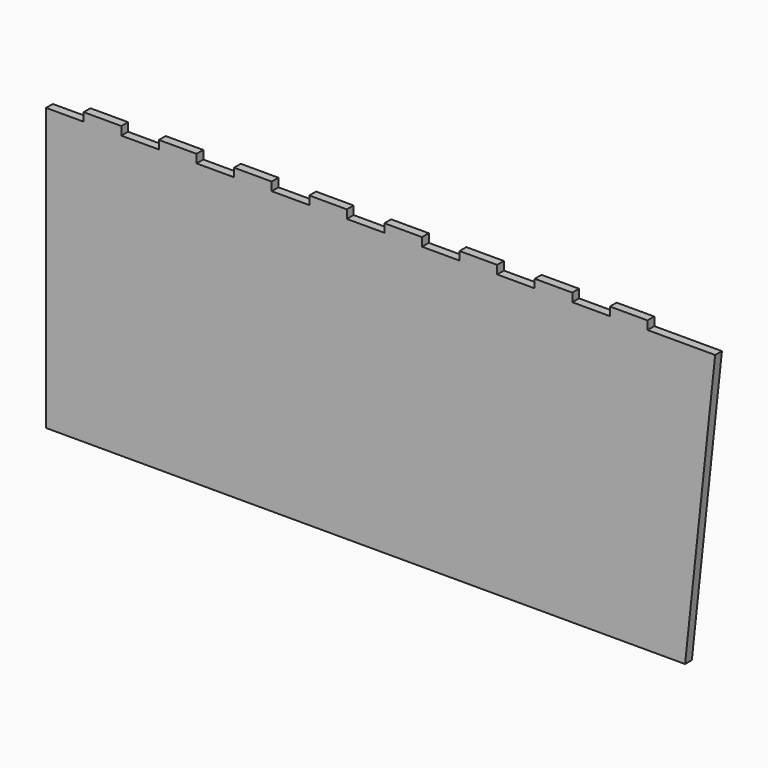
from build123d import *

# Parameters (mm, degrees)
F1_DEPTH = 3


# Not quite as in the source:
# - ends of sketch curves that miss each other by under 0.0002 mm in the source are joined


with BuildPart() as f1:
    # F0 (on Front) → F1 (new body)
    with BuildSketch(Plane.XZ):
        Polygon((-86.6666681571, 50), (-100.0000014901, 50), (-100.0000014901, 53.0000007451), (-113.3729092283, 53.0000007451), (-113.3729092283, 50.0000007451), (-126.7062425613, 50.0000007451), (-126.7062425613, -50), (100, -50), (110.67250236, 50), (86.6666611759, 50), (86.6666611759, 53), (73.3333278429, 53), (73.3333278429, 50), (59.9999951759, 50), (59.9999951759, 53), (46.6666618429, 53), (46.6666618429, 50), (33.3333291759, 50), (33.3333291759, 53), (19.9999958429, 53), (19.9999958429, 50), (6.6666631759, 50), (6.6666631759, 53), (-6.6666701571, 53), (-6.6666701571, 50), (-20.0000028241, 50), (-20.0000028241, 53), (-33.3333361571, 53), (-33.3333361571, 50), (-46.6666688241, 50), (-46.6666688241, 53), (-60.0000021571, 53), (-60.0000021571, 50), (-73.3333348241, 50), (-73.3333348241, 53), (-86.6666681571, 53), align=None)
    extrude(amount=F1_DEPTH)


solid = f1.part
